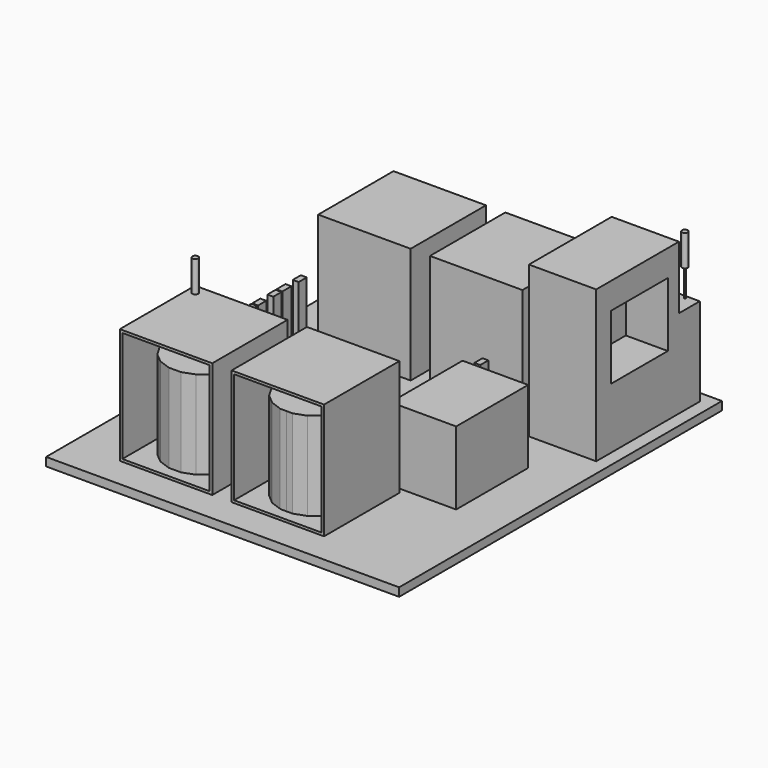
from build123d import *

# Parameters (mm, degrees)
F0_W      = 1100
F0_H      = 1120
F1_DEPTH  = 1380
F0_W_2    = 800
F0_H_2    = 1230
F2_DEPTH  = 1800
F3_DEPTH  = 1050
F0_W_3    = 70
F0_H_3    = 120
F4_DEPTH  = 850
F0_H_4    = 122.0874786377
F0_H_5    = 135
F5_T      = -30
F5_2_T    = -30
F5_3_T    = -30
F5_4_T    = -30
F7_DEPTH  = 1050
F0_W_4    = 620.9681331739
F0_H_6    = 223.0965256691
F0_H_7    = 846.9034743309
F0_W_5    = 159.0318668261
F8_DEPTH  = 870
F9_T      = -50
F0_R      = 500
F10_DEPTH = 100
F11_DEPTH = 50
F12_R     = 35
F13_DEPTH = 370
F14_R     = 10
F15_DEPTH = 350
F16_W     = 842.3538208008
F16_H     = 764.7948861122
F17_DEPTH = 500


with BuildPart() as f1:
    # F0 (on Top) → F1 (new body)
    with BuildSketch(Plane.XY):
        with Locations((-1721.9454687461, 3475.8938026428)):
            Rectangle(F0_W, F0_H)
    extrude(amount=F1_DEPTH)

    # F5#4
    f5_4_openings = [f1.faces().sort_by_distance(p)[0] for p in [
        (-1721.945469, 4035.893803, 690),
    ]]
    offset(amount=F5_4_T, openings=f5_4_openings)


with BuildPart() as f1b:
    # F0 (on Top) → F1, piece 2 (new body)
    with BuildSketch(Plane.XY):
        with Locations((-3051.9454687461, 3475.8938026428)):
            Rectangle(F0_W, F0_H)
    extrude(amount=F1_DEPTH)

    # F5#3
    f5_3_openings = [f1b.faces().sort_by_distance(p)[0] for p in [
        (-3051.945469, 4035.893803, 690),
    ]]
    offset(amount=F5_3_T, openings=f5_3_openings)


with BuildPart() as f1c:
    # F0 (on Top) → F1, piece 3 (new body)
    with BuildSketch(Plane.XY):
        with Locations((-1721.9454687461, 525.8938026428)):
            Rectangle(F0_W, F0_H)
    extrude(amount=F1_DEPTH)

    # F5
    f5_openings = [f1c.faces().sort_by_distance(p)[0] for p in [
        (-1721.945469, -34.106197, 690),
    ]]
    offset(amount=F5_T, openings=f5_openings)

    # F6 (on face) → F7 (join)
    with BuildSketch(Plane.XY.offset(30)):
        Polygon((-1721.9454687461, 510.8938026428), (-1721.9454687461, 95.6590033894), (-1650.902164665, 95.2874173432), (-1513.0408446776, 144.6497902694), (-1400.3765054567, 238.1865962738), (-1326.4981290611, 364.6159160961), (-1300.3165380126, 508.6885078675), (-1300.6935087061, 510.8938026428), align=None)
        Polygon((-1797.3323556121, 96.0533081811), (-1721.9454687461, 95.6590033894), (-1721.9454687461, 510.8938026428), (-2143.1974287861, 510.8938026428), (-2118.9013189014, 368.7605145501), (-2046.34950435, 241.56530389), (-1934.6697754111, 146.8550850447), align=None)
        Polygon((-2143.5743994797, 513.0990974181), (-2143.1974287861, 510.8938026428), (-1721.9454687461, 510.8938026428), (-1721.9454687461, 926.1286018963), (-1792.9887728273, 926.5001879424), (-1930.8500928147, 877.1378150162), (-2043.5144320355, 783.6010090118), (-2117.3928084312, 657.1716891896), align=None)
        Polygon((-1721.9454687461, 926.1286018963), (-1721.9454687461, 510.8938026428), (-1300.6935087061, 510.8938026428), (-1324.9896185908, 653.0270907356), (-1397.5414331422, 780.2223013957), (-1509.2211620811, 874.9325202409), (-1646.5585818802, 925.7342971045), align=None)
    extrude(amount=F7_DEPTH)


with BuildPart() as f1d:
    # F0 (on Top) → F1, piece 4 (new body)
    with BuildSketch(Plane.XY):
        with Locations((-3051.9454687461, 525.8938026428)):
            Rectangle(F0_W, F0_H)
    extrude(amount=F1_DEPTH)

    # F5#2
    f5_2_openings = [f1d.faces().sort_by_distance(p)[0] for p in [
        (-3051.945469, -34.106197, 690),
    ]]
    offset(amount=F5_2_T, openings=f5_2_openings)

    # F12 (on face) → F13 (join)
    with BuildSketch(Plane.XY.offset(1380)):
        with Locations((-3512.1169090271, 975.8208394051)):
            Circle(F12_R)
    extrude(amount=F13_DEPTH)


with BuildPart() as f2:
    # F0 (on Top) → F2 (new body)
    with BuildSketch(Plane.XY):
        with Locations((-541.1582165956, 3339.161863327)):
            Rectangle(F0_W_2, F0_H_2)
    extrude(amount=F2_DEPTH)

    # F0 (on Top) → F3 (join)
    with BuildSketch(Plane.XY):
        Polygon((-941.1582165956, 3954.161863327), (-141.1582165956, 3954.161863327), (-141.1582165956, 4264.161863327), (-1101.1582165956, 4264.161863327), (-1101.1582165956, 3954.161863327), align=None)
    extrude(amount=F3_DEPTH)

    # F16 (on face) → F17 (cut)
    with BuildSketch(Plane.YZ.offset(-141.1582165956)):
        with Locations((3368.0732250214, 1104.4473350048)):
            Rectangle(F16_W, F16_H)
    extrude(amount=-F17_DEPTH, mode=Mode.SUBTRACT)


with BuildPart() as f4:
    # F0 (on Top) → F4 (new body)
    with BuildSketch(Plane.XY):
        with Locations((-3566.9454687461, 2598.177728653)):
            Rectangle(F0_W_3, F0_H_3)
    extrude(amount=F4_DEPTH)


with BuildPart() as f4b:
    # F0 (on Top) → F4, piece 2 (new body)
    with BuildSketch(Plane.XY):
        Polygon((-3531.9454687461, 2430.3176593781), (-3601.9454687461, 2430.3176593781), (-3601.9454687461, 2383.2371234894), (-3601.9454687461, 2295.3176593781), (-3531.9454687461, 2295.3176593781), align=None)
    extrude(amount=F4_DEPTH)


with BuildPart() as f4c:
    # F0 (on Top) → F4, piece 3 (new body)
    with BuildSketch(Plane.XY):
        with Locations((-3566.9454687461, 2221.3613986969)):
            Rectangle(F0_W_3, F0_H_4)
    extrude(amount=F4_DEPTH)


with BuildPart() as f4d:
    # F0 (on Top) → F4, piece 4 (new body)
    with BuildSketch(Plane.XY):
        Polygon((-3601.9454687461, 2000.8938026428), (-3601.9454687461, 1935.2961778641), (-3531.9454687461, 1933.9606761932), (-3531.9454687461, 2056.5693569183), (-3601.9454687461, 2056.5693569183), align=None)
    extrude(amount=F4_DEPTH)


with BuildPart() as f4e:
    # F0 (on Top) → F4, piece 5 (new body)
    with BuildSketch(Plane.XY):
        with Locations((-3566.9454687461, 1854.0693569183)):
            Rectangle(F0_W_3, F0_H_5)
    extrude(amount=F4_DEPTH)


with BuildPart() as f4f:
    # F0 (on Top) → F4, piece 6 (new body)
    with BuildSketch(Plane.XY):
        with Locations((-1206.9454687461, 2348.8567447662)):
            Rectangle(F0_W_3, F0_H_3)
    extrude(amount=F4_DEPTH)


with BuildPart() as f7:
    # F6 (on face) → F7, piece 2 (new body)
    with BuildSketch(Plane.XY.offset(30)):
        Polygon((-1721.9454687461, 3075.6590033894), (-1721.9454687461, 3490.8938026428), (-2143.1974287861, 3490.8938026428), (-2143.5743994797, 3488.6885078675), (-2117.3928084312, 3344.6159160961), (-2043.5144320355, 3218.1865962738), (-1930.8500928147, 3124.6497902694), (-1792.9887728273, 3075.2874173432), align=None)
        Polygon((-1300.6935087061, 3490.8938026428), (-1721.9454687461, 3490.8938026428), (-1721.9454687461, 3075.6590033894), (-1646.5585818802, 3076.0533081811), (-1509.2211620811, 3126.8550850447), (-1397.5414331422, 3221.56530389), (-1324.9896185908, 3348.7605145501), align=None)
        Polygon((-1650.902164665, 3906.5001879424), (-1721.9454687461, 3906.1286018963), (-1721.9454687461, 3490.8938026428), (-1300.6935087061, 3490.8938026428), (-1300.3165380126, 3493.0990974181), (-1326.4981290611, 3637.1716891896), (-1400.3765054567, 3763.6010090118), (-1513.0408446776, 3857.1378150162), align=None)
        Polygon((-1721.9454687461, 3490.8938026428), (-1721.9454687461, 3906.1286018963), (-1797.3323556121, 3905.7342971045), (-1934.6697754111, 3854.9325202409), (-2046.34950435, 3760.2223013957), (-2118.9013189014, 3633.0270907356), (-2143.1974287861, 3490.8938026428), align=None)
    extrude(amount=F7_DEPTH)


with BuildPart() as f7b:
    # F6 (on face) → F7, piece 3 (new body)
    with BuildSketch(Plane.XY.offset(30)):
        Polygon((-2839.2211620811, 3854.9325202409), (-2976.5585818802, 3905.7342971045), (-3051.9454687461, 3906.1286018963), (-3051.9454687461, 3490.8938026428), (-2630.6935087061, 3490.8938026428), (-2654.9896185908, 3633.0270907356), (-2727.5414331422, 3760.2223013957), align=None)
        Polygon((-2630.6935087061, 3490.8938026428), (-3051.9454687461, 3490.8938026428), (-3051.9454687461, 3075.6590033894), (-2980.902164665, 3075.2874173432), (-2843.0408446776, 3124.6497902694), (-2730.3765054567, 3218.1865962738), (-2656.4981290611, 3344.6159160961), (-2630.3165380126, 3488.6885078675), align=None)
        Polygon((-3051.9454687461, 3075.6590033894), (-3051.9454687461, 3490.8938026428), (-3473.1974287861, 3490.8938026428), (-3448.9013189014, 3348.7605145501), (-3376.34950435, 3221.56530389), (-3264.6697754111, 3126.8550850447), (-3127.3323556121, 3076.0533081811), align=None)
        Polygon((-3051.9454687461, 3490.8938026428), (-3051.9454687461, 3906.1286018963), (-3122.9887728273, 3906.5001879424), (-3260.8500928147, 3857.1378150162), (-3373.5144320355, 3763.6010090118), (-3447.3928084312, 3637.1716891896), (-3473.5743994797, 3493.0990974181), (-3473.1974287861, 3490.8938026428), align=None)
    extrude(amount=F7_DEPTH)


with BuildPart() as f7c:
    # F6 (on face) → F7, piece 4 (new body)
    with BuildSketch(Plane.XY.offset(30)):
        Polygon((-2976.5585818802, 96.0533081811), (-2839.2211620811, 146.8550850447), (-2727.5414331422, 241.56530389), (-2654.9896185908, 368.7605145501), (-2630.3165380126, 513.0990974181), (-2656.4981290611, 657.1716891896), (-2730.3765054567, 783.6010090118), (-2843.0408446776, 877.1378150162), (-2980.902164665, 926.5001879424), (-3127.3323556121, 925.7342971045), (-3264.6697754111, 874.9325202409), (-3376.34950435, 780.2223013957), (-3448.9013189014, 653.0270907356), (-3473.5743994797, 508.6885078675), (-3447.3928084312, 364.6159160961), (-3373.5144320355, 238.1865962738), (-3260.8500928147, 144.6497902694), (-3122.9887728273, 95.2874173432), align=None)
    extrude(amount=F7_DEPTH)


with BuildPart() as f8:
    # F0 (on Top) → F8 (new body)
    with BuildSketch(Plane.XY):
        with Locations((-861.4614021592, 2112.4420654774)):
            Rectangle(F0_W_4, F0_H_6)
        with Locations((-861.4614021592, 1577.4420654774)):
            Rectangle(F0_W_4, F0_H_7)
        with Locations((-1251.4614021592, 1577.4420654774)):
            Rectangle(F0_W_5, F0_H_7)
        with Locations((-1251.4614021592, 2112.4420654774)):
            Rectangle(F0_W_5, F0_H_6)
    extrude(amount=F8_DEPTH)

    # F9
    f9_openings = [f8.faces().sort_by_distance(p)[0] for p in [
        (-1330.977336, 1688.990328, 435),
    ]]
    offset(amount=F9_T, openings=f9_openings)


with BuildPart() as f10:
    # F0 (on Top) → F10 (new body)
    with BuildSketch(Plane.XY):
        Polygon((-3604.0337085724, 4400.8938026428), (-4186.9454687461, 4400.8938026428), (-4186.9454687461, -399.1061973572), (13.0545312539, -399.1061973572), (13.0545312539, 2000.8938026428), (13.0545312539, 4400.8938026428), (-1092.3580169678, 4400.8938026428), (-2192.3580169678, 4400.8938026428), (-2504.0337085724, 4400.8938026428), align=None)
        Polygon((-550.9773355722, 2223.9903283119), (-550.9773355722, 2000.8938026428), (-550.9773355722, 1153.9903283119), (-1171.9454687461, 1153.9903283119), (-1171.9454687461, 1085.8938026428), (-1171.9454687461, -34.1061973572), (-2271.9454687461, -34.1061973572), (-2271.9454687461, 1085.8938026428), (-2501.9454687461, 1085.8938026428), (-2501.9454687461, -34.1061973572), (-3601.9454687461, -34.1061973572), (-3601.9454687461, 1085.8938026428), (-3601.9454687461, 1786.5693569183), (-3601.9454687461, 1921.5693569183), (-3601.9454687461, 1935.2961778641), (-3601.9454687461, 2000.8938026428), (-3601.9454687461, 2056.5693569183), (-3601.9454687461, 2160.3176593781), (-3601.9454687461, 2282.4051380157), (-3601.9454687461, 2295.3176593781), (-3601.9454687461, 2383.2371234894), (-3601.9454687461, 2430.3176593781), (-3601.9454687461, 2538.177728653), (-3601.9454687461, 2658.177728653), (-3601.9454687461, 2915.8938026428), (-3601.9454687461, 4035.8938026428), (-2501.9454687461, 4035.8938026428), (-2501.9454687461, 2915.8938026428), (-2386.9454687461, 2915.8938026428), (-2271.9454687461, 2915.8938026428), (-2271.9454687461, 4035.8938026428), (-1171.9454687461, 4035.8938026428), (-1171.9454687461, 2915.8938026428), (-1171.9454687461, 2408.8567447662), (-1171.9454687461, 2288.8567447662), (-1171.9454687461, 2223.9903283119), align=None, mode=Mode.SUBTRACT)
        Polygon((-141.1582165956, 3954.161863327), (-141.1582165956, 2724.161863327), (-941.1582165956, 2724.161863327), (-941.1582165956, 3954.161863327), (-1101.1582165956, 3954.161863327), (-1101.1582165956, 4264.161863327), (-141.1582165956, 4264.161863327), align=None, mode=Mode.SUBTRACT)
        Polygon((-1330.9773355722, 1153.9903283119), (-1330.9773355722, 2000.8938026428), (-1330.9773355722, 2223.9903283119), (-1171.9454687461, 2223.9903283119), (-1171.9454687461, 2288.8567447662), (-1241.9454687461, 2288.8567447662), (-1241.9454687461, 2408.8567447662), (-1171.9454687461, 2408.8567447662), (-1171.9454687461, 2915.8938026428), (-2271.9454687461, 2915.8938026428), (-2386.9454687461, 2915.8938026428), (-2501.9454687461, 2915.8938026428), (-3601.9454687461, 2915.8938026428), (-3601.9454687461, 2658.177728653), (-3531.9454687461, 2658.177728653), (-3531.9454687461, 2538.177728653), (-3601.9454687461, 2538.177728653), (-3601.9454687461, 2430.3176593781), (-3531.9454687461, 2430.3176593781), (-3531.9454687461, 2295.3176593781), (-3531.9454687461, 2282.4051380157), (-3531.9454687461, 2160.3176593781), (-3601.9454687461, 2160.3176593781), (-3601.9454687461, 2056.5693569183), (-3531.9454687461, 2056.5693569183), (-3531.9454687461, 1933.9606761932), (-3531.9454687461, 1921.5693569183), (-3531.9454687461, 1786.5693569183), (-3601.9454687461, 1786.5693569183), (-3601.9454687461, 1085.8938026428), (-2501.9454687461, 1085.8938026428), (-2271.9454687461, 1085.8938026428), (-1171.9454687461, 1085.8938026428), (-1171.9454687461, 1153.9903283119), align=None)
        with Locations((-2386.9454687461, 2000.8938026428)):
            Circle(F0_R, mode=Mode.SUBTRACT)
        with Locations((-3051.9454687461, 525.8938026428)):
            Rectangle(F0_W, F0_H)
        with Locations((-1721.9454687461, 525.8938026428)):
            Rectangle(F0_W, F0_H)
        with Locations((-3051.9454687461, 3475.8938026428)):
            Rectangle(F0_W, F0_H)
        with Locations((-1721.9454687461, 3475.8938026428)):
            Rectangle(F0_W, F0_H)
        with Locations((-541.1582165956, 3339.161863327)):
            Rectangle(F0_W_2, F0_H_2)
        with Locations((-2386.9454687461, 2000.8938026428)):
            Circle(F0_R)
        with Locations((-861.4614021592, 1577.4420654774)):
            Rectangle(F0_W_4, F0_H_7)
        Polygon((-941.1582165956, 3954.161863327), (-141.1582165956, 3954.161863327), (-141.1582165956, 4264.161863327), (-1101.1582165956, 4264.161863327), (-1101.1582165956, 3954.161863327), align=None)
        with Locations((-861.4614021592, 2112.4420654774)):
            Rectangle(F0_W_4, F0_H_6)
        with Locations((-1251.4614021592, 1577.4420654774)):
            Rectangle(F0_W_5, F0_H_7)
        with Locations((-1251.4614021592, 2112.4420654774)):
            Rectangle(F0_W_5, F0_H_6)
        Polygon((-3531.9454687461, 2430.3176593781), (-3601.9454687461, 2430.3176593781), (-3601.9454687461, 2383.2371234894), (-3601.9454687461, 2295.3176593781), (-3531.9454687461, 2295.3176593781), align=None)
        with Locations((-3566.9454687461, 1854.0693569183)):
            Rectangle(F0_W_3, F0_H_5)
        with Locations((-3566.9454687461, 2221.3613986969)):
            Rectangle(F0_W_3, F0_H_4)
        Polygon((-3601.9454687461, 2000.8938026428), (-3601.9454687461, 1935.2961778641), (-3531.9454687461, 1933.9606761932), (-3531.9454687461, 2056.5693569183), (-3601.9454687461, 2056.5693569183), align=None)
        with Locations((-3566.9454687461, 2598.177728653)):
            Rectangle(F0_W_3, F0_H_3)
        with Locations((-1206.9454687461, 2348.8567447662)):
            Rectangle(F0_W_3, F0_H_3)
    extrude(amount=-F10_DEPTH)

    # F0 (on Top) → F11 (join)
    with BuildSketch(Plane.XY):
        with Locations((-2386.9454687461, 2000.8938026428)):
            Circle(F0_R)
    extrude(amount=F11_DEPTH)


with BuildPart() as f13:
    # F12 (on face) → F13, piece 2 (new body)
    with BuildSketch(Plane.XY.offset(1380)):
        with Locations((-287.6563072205, 4227.4084091187)):
            Circle(F12_R)
    extrude(amount=F13_DEPTH)


with BuildPart() as f15:
    # F14 (on face) → F15 (new body)
    with BuildSketch(Plane(origin=(0, 0, 1380), x_dir=(1, 0, 0), z_dir=(0, 0, -1))):
        with Locations((-287.6563072205, -4227.4084091187)):
            Circle(F14_R)
    extrude(amount=F15_DEPTH)


solid = Compound([f1.part, f1b.part, f1c.part, f1d.part, f2.part, f4.part, f4b.part, f4c.part, f4d.part, f4e.part, f4f.part, f7.part, f7b.part, f7c.part, f8.part, f10.part, f13.part, f15.part])
